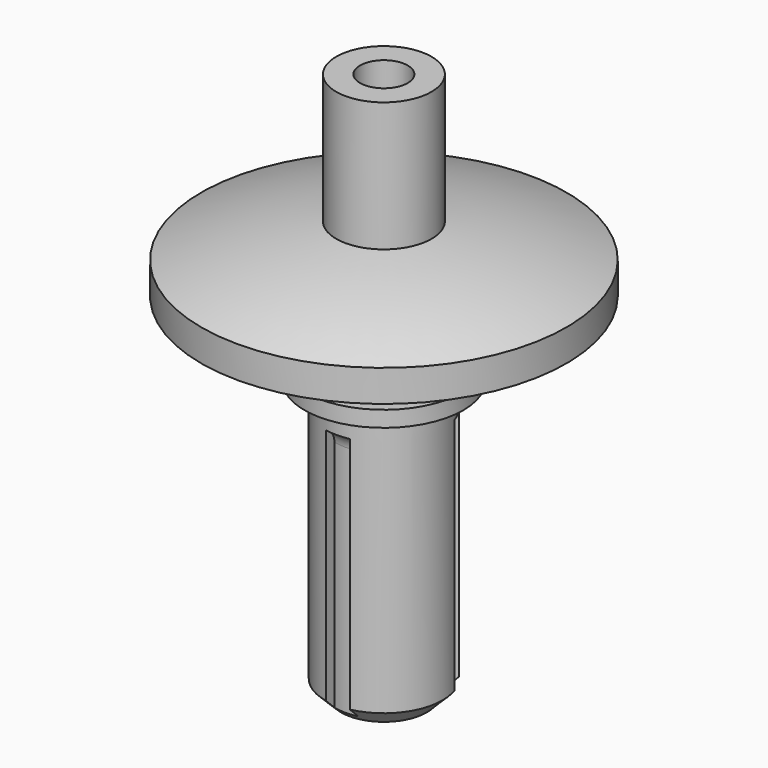
from build123d import *

# Parameters (mm, degrees)
F0_R        = 3.7
F1_DEPTH    = 17.5
F3_DEPTH    = 16
F4_T2_ANGLE = 116.4603484981
F4_T4_ANGLE = 116.4603484981
F4_T6_ANGLE = 116.4603484981
F5_T2_ANGLE = 176.2935685117
F5_T4_ANGLE = 176.2935685117
F5_T6_ANGLE = 58.1290115734
F5_T8_ANGLE = 118.1404591149
F6_R        = 5
F7_DEPTH    = 1
F8_R        = 3
F9_DEPTH    = 16
F14_DEPTH   = 25
F15_R       = 1.5
F16_DEPTH   = 25


# Not quite as in the source:
# - a fillet or chamfer that OpenCascade refuses, or shapes differently, is made with other operations: its cross-section is extruded or revolved along the edge and cut away or added


with BuildPart() as f1:
    # F0 (on Top) → F1 (new body)
    with BuildSketch(Plane.XY):
        Circle(F0_R)
    extrude(amount=-F1_DEPTH)

    # F2 (on face) → F3 (cut)
    with BuildSketch(Plane(origin=(0, 0, -17.5), x_dir=(1, 0, 0), z_dir=(0, 0, -1))):
        with BuildLine():
            ThreePointArc((-2.1852734229, -2.1276936027), (-2.6413774815, -1.525), (-2.9352734229, -0.8286554971))
            Line((-2.9352734229, -0.8286554971), (-3.5127738924, -1.1620755486))
            ThreePointArc((-3.5127738924, -1.1620755486), (-3.204293994, -1.85), (-2.7627738924, -2.4611136543))
            Line((-2.7627738924, -2.4611136543), (-2.1852734229, -2.1276936027))
        make_face()
        with BuildLine():
            Line((-0.75, 3.6231892029), (-0.75, 2.9563490998))
            ThreePointArc((-0.75, 2.9563490998), (0, 3.05), (0.75, 2.9563490998))
            Line((0.75, 2.9563490998), (0.75, 3.6231892029))
            ThreePointArc((0.75, 3.6231892029), (0, 3.7), (-0.75, 3.6231892029))
        make_face()
        with BuildLine():
            Line((2.1852734229, -2.1276936027), (2.7627738924, -2.4611136543))
            ThreePointArc((2.7627738924, -2.4611136543), (3.204293994, -1.85), (3.5127738924, -1.1620755486))
            Line((3.5127738924, -1.1620755486), (2.9352734229, -0.8286554971))
            ThreePointArc((2.9352734229, -0.8286554971), (2.6413774815, -1.525), (2.1852734229, -2.1276936027))
        make_face()
    extrude(amount=-F3_DEPTH, mode=Mode.SUBTRACT)

    # F4: fillet of radius 1 on 3 edges, made by hand

    # F4_s1 → F4_t2 (revolve)
    with BuildSketch(Plane(origin=(0, 0, 0), x_dir=(0, 0, 1), z_dir=(-0.473014829, -0.8810544657, 0))):
        with BuildLine():
            ThreePointArc((-1.5, -3.7), (-1.8666619872, -3.2284161637), (-2.4367496998, -3.05))
            Line((-2.4367496998, -3.05), (-1.5, -3.05))
            Line((-1.5, -3.05), (-1.5, -3.7))
        make_face()
    revolve(axis=Axis((0, 0, -1.5), (0, 0, 1)), revolution_arc=F4_T2_ANGLE)

    # F4_s3 → F4_t4 (revolve)
    with BuildSketch(Plane(origin=(0, 0, 0), x_dir=(0, 0, 1), z_dir=(-0.526508135, 0.8501700911, 0))):
        with BuildLine():
            ThreePointArc((-1.5, -3.7), (-1.8666619872, -3.2284161637), (-2.4367496998, -3.05))
            Line((-2.4367496998, -3.05), (-1.5, -3.05))
            Line((-1.5, -3.05), (-1.5, -3.7))
        make_face()
    revolve(axis=Axis((0, 0, -1.5), (0, 0, 1)), revolution_arc=F4_T4_ANGLE)

    # F4_s5 → F4_t6 (revolve)
    with BuildSketch(Plane(origin=(0, 0, 0), x_dir=(0, 0, 1), z_dir=(0.9995229639, 0.0308843746, 0))):
        with BuildLine():
            ThreePointArc((-1.5, -3.7), (-1.8666619872, -3.2284161637), (-2.4367496998, -3.05))
            Line((-2.4367496998, -3.05), (-1.5, -3.05))
            Line((-1.5, -3.05), (-1.5, -3.7))
        make_face()
    revolve(axis=Axis((0, 0, -1.5), (0, 0, 1)), revolution_arc=F4_T6_ANGLE)

    # F5: chamfer of 1 on 4 edges, made by hand

    # F5_s1 → F5_t2 (revolve, cut)
    with BuildSketch(Plane(origin=(0, 0, 0), x_dir=(0, 0, 1), z_dir=(0.8494028952, 0.5277449399, 0))):
        Polygon((-16.5, -3.7), (-17.5, -2.7), (-17.5, -3.7), align=None)
    revolve(axis=Axis((0, 0, -17.5), (0, 0, 1)), revolution_arc=F5_T2_ANGLE, mode=Mode.SUBTRACT)

    # F5_s3 → F5_t4 (revolve, cut)
    with BuildSketch(Plane(origin=(0, 0, 0), x_dir=(0, 0, 1), z_dir=(0.032339077, -0.9994769553, 0))):
        Polygon((-16.5, -3.7), (-17.5, -2.7), (-17.5, -3.7), align=None)
    revolve(axis=Axis((0, 0, -17.5), (0, 0, 1)), revolution_arc=F5_T4_ANGLE, mode=Mode.SUBTRACT)

    # F5_s5 → F5_t6 (revolve, cut)
    with BuildSketch(Plane.XZ):
        Polygon((3.7, -16.5), (2.7, -17.5), (3.7, -17.5), align=None)
    revolve(axis=Axis((0, 0, -17.5), (0, 0, 1)), revolution_arc=F5_T6_ANGLE, mode=Mode.SUBTRACT)

    # F5_s7 → F5_t8 (revolve, cut)
    with BuildSketch(Plane(origin=(0, 0, 0), x_dir=(0, 0, 1), z_dir=(-0.8817940435, 0.471634673, 0))):
        Polygon((-16.5, -3.7), (-17.5, -2.7), (-17.5, -3.7), align=None)
    revolve(axis=Axis((0, 0, -17.5), (0, 0, 1)), revolution_arc=F5_T8_ANGLE, mode=Mode.SUBTRACT)

    # F6 (on face) → F7 (join)
    with BuildSketch(Plane.XY):
        Circle(F6_R)
    extrude(amount=F7_DEPTH)

    # F8 (on face) → F9 (join)
    with BuildSketch(Plane.XY.offset(1)):
        Circle(F8_R)
    extrude(amount=F9_DEPTH)

    # F10 (on Right) → F12 (revolve)
    with BuildSketch(Plane.YZ):
        with BuildLine():
            Line((0, 8), (0, 9))
            ThreePointArc((0, 9), (-5.863059775, 8.4214977538), (-11.5, 6.708302005))
            Line((-11.5, 6.708302005), (-11.5, 4.708302005))
            ThreePointArc((-11.5, 4.708302005), (-5.9157247408, 6.9331331941), (0, 8))
        make_face()
    revolve(axis=Axis((0, 0, 8.2032438368), (0, 0, 1)))

    # F13 (on Right) → F14 (cut)
    with BuildSketch(Plane.YZ):
        with BuildLine():
            ThreePointArc((2, 3.5), (1.8535533906, 3.8535533906), (1.5, 4))
            Line((1.5, 4), (-1.5, 4))
            ThreePointArc((-1.5, 4), (-1.8535533906, 3.8535533906), (-2, 3.5))
            Line((-2, 3.5), (-2, 2.5))
            ThreePointArc((-2, 2.5), (-1.8535533906, 2.1464466094), (-1.5, 2))
            Line((-1.5, 2), (1.5, 2))
            ThreePointArc((1.5, 2), (1.8535533906, 2.1464466094), (2, 2.5))
            Line((2, 2.5), (2, 3.5))
        make_face()
    extrude(amount=-F14_DEPTH, mode=Mode.SUBTRACT)

    # F15 (on face) → F16 (cut)
    with BuildSketch(Plane.XY.offset(17)):
        Circle(F15_R)
    extrude(amount=-F16_DEPTH, mode=Mode.SUBTRACT)


solid = f1.part
